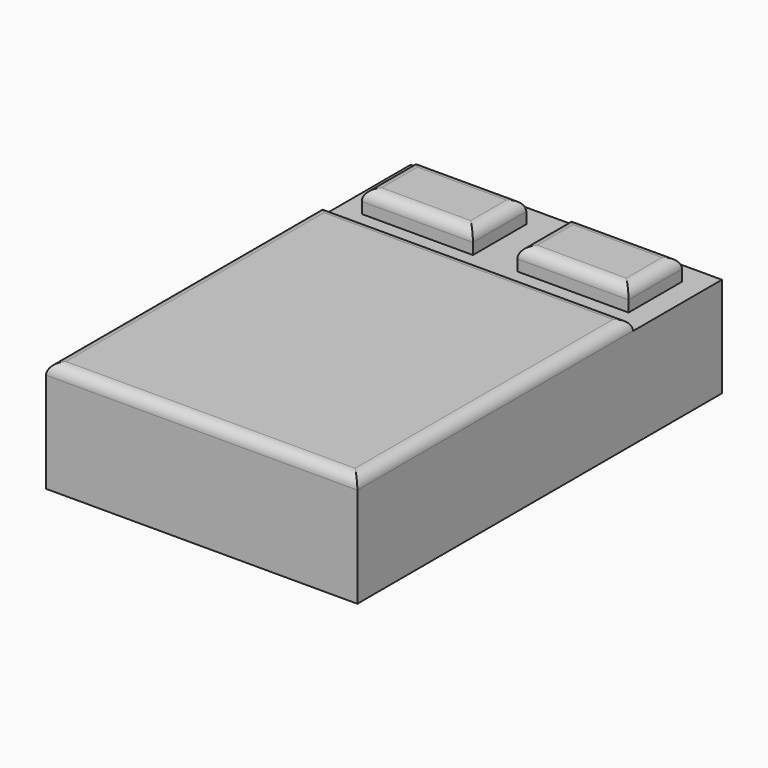
from build123d import *

# Parameters (mm, degrees)
F0_W     = 28
F0_H     = 10
F0_W_2   = 10
F0_H_2   = 6
F0_H_3   = 31
F1_DEPTH = 9
F2_DEPTH = 1
F3_DEPTH = 2
F4_R     = 0.99999


# Not quite as in the source:
# - a fillet or chamfer is up to 0.001 mm smaller than in the source, because OpenCascade refuses the exact size


with BuildPart() as f1:
    # F0 (on Top) → F1 (new body)
    with BuildSketch(Plane.XY):
        with Locations((14, 36)):
            Rectangle(F0_W, F0_H)
        with Locations((7, 36)):
            Rectangle(F0_W_2, F0_H_2, mode=Mode.SUBTRACT)
        with Locations((21, 36)):
            Rectangle(F0_W_2, F0_H_2, mode=Mode.SUBTRACT)
        with Locations((7, 36)):
            Rectangle(F0_W_2, F0_H_2)
        with Locations((21, 36)):
            Rectangle(F0_W_2, F0_H_2)
        with Locations((14, 15.5)):
            Rectangle(F0_W, F0_H_3)
    extrude(amount=-F1_DEPTH)

    # F0 (on Top) → F2 (join)
    with BuildSketch(Plane.XY):
        with Locations((14, 15.5)):
            Rectangle(F0_W, F0_H_3)
    extrude(amount=F2_DEPTH)

    # F0 (on Top) → F3 (join)
    with BuildSketch(Plane.XY):
        with Locations((7, 36)):
            Rectangle(F0_W_2, F0_H_2)
        with Locations((21, 36)):
            Rectangle(F0_W_2, F0_H_2)
    extrude(amount=F3_DEPTH)

    # F4 (radius 1 in the source; OpenCascade refuses exactly that, so slightly less here)
    f4_edges = [f1.edges().sort_by_distance(p)[0] for p in [
        (12, 36, 2),
        (7, 39, 2),
        (2, 36, 2),
        (7, 33, 2),
        (21, 39, 2),
        (16, 36, 2),
        (21, 33, 2),
        (26, 36, 2),
        (0, 15.5, 1),
        (14, 0, 1),
        (28, 15.5, 1),
        (14, 31, 1),
    ]]
    fillet(f4_edges, radius=F4_R)


solid = f1.part
